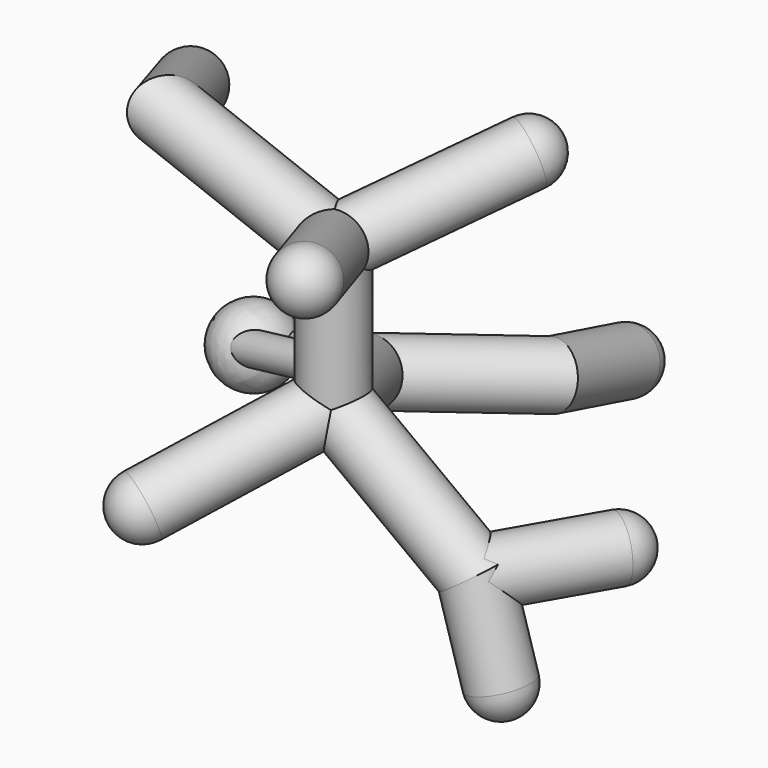
from build123d import *

# Parameters (mm, degrees)
F9_R  = 6
F13_R = 6
F18_R = 6
F26_R = 6
F29_R = 6
F31_R = 6
F34_R = 3


with BuildPart() as f11:
    # F11: sweep along a path in F7, F4
    with BuildLine(Plane(origin=(-5.0749581016, 8.7900852782, 27.9244028222), x_dir=(0.9853046871, 0.051285676, 0.1629246852), z_dir=(0.1708059531, -0.295844589, -0.9398411066))) as f11_path:
        Line((2.0467480645, -75.1046538353), (6.1499904841, -45.6850528717))
        Line((6.1499904841, -45.6850528717), (-12.6624797904, -23.3359215656))
        Line((-12.6624797904, -23.3359215656), (5.1506484929, 9.4922267384))
    with BuildLine(Plane.XZ) as f11_path_2:
        Line((0, 31.6136777401), (0, 58.9116849005))
    # F9 (on line) → F11 (sweep)
    with BuildSketch(Plane(origin=(-10.0857183749, 69.480148269, -23.7040351701), x_dir=(-0.9906942747, -0.1288157724, 0.0439471371), z_dir=(-0.1361060398, 0.9376295745, -0.3198842398))):
        with Locations((-7.0934403418, 31.4051011688)):
            Circle(F9_R)
    sweep(path=f11_path.line + f11_path_2.line, transition=Transition.RIGHT)

    # F14: sweep along a path in F4, F10
    with BuildLine(Plane.XZ) as f14_path:
        Line((34.7157008946, -12.1698062867), (27.8801377863, 10.8416592702))
        Line((27.8801377863, 10.8416592702), (0, 31.6136777401))
    with BuildLine(Plane(origin=(0, 0, 0), x_dir=(-0.5, -0.8660254038, 0), z_dir=(-0.8660254038, 0.5, 0))) as f14_path_2:
        Line((0, 31.6136777401), (37.2237116098, 17.5120830536))
    # F13 (on line) → F14 (sweep)
    with BuildSketch(Plane(origin=(6.1368140533, 0, -20.6591736452), x_dir=(0.9586010028, 0, 0.2847527305), z_dir=(0.2847527305, 0, -0.9586010028))):
        with Locations((29.8131201191, 0)):
            Circle(F13_R)
    sweep(path=f14_path.line + f14_path_2.line, transition=Transition.RIGHT)

    # F19: sweep along a path in F16
    with BuildLine(Plane.XY.offset(10.8416592702)) as f19_path:
        Line((27.8801377863, 0), (42.7882038549, 25.8215278734))
    # F18 (on line) → F19 (sweep)
    with BuildSketch(Plane(origin=(21.8781005152, 37.8939816654, 0), x_dir=(-0.8660254038, 0.5, 0), z_dir=(0.5, 0.8660254038, 0))):
        with Locations((-24.1449075839, 10.8416592702)):
            Circle(F18_R)
    sweep(path=f19_path.line)

    # F27: sweep along a path in F27_path
    with BuildLine(Plane(origin=(0, 0, 58.9116849005), x_dir=(0.8527843216, 0, 0.5222632486), z_dir=(0.5222626897, 0.0014629567, -0.852783409))) as f27_path:
        Line((20.2068447746, 29.8864215955), (0, 0))
        Line((0, 0), (22.3578653078, -32.9804275589))
    # F26 (on line) → F27 (sweep)
    with BuildSketch(Plane(origin=(25.4681834782, -44.1121877608, 15.5215822052), x_dir=(0.8782037706, 0.4511717321, -0.1587520249), z_dir=(0.4782866685, -0.8284168104, 0.2914917685))):
        with Locations((-9.352349266, 55.5718749217)):
            Circle(F26_R)
    sweep(path=f27_path.line, transition=Transition.RIGHT)

    # F30: sweep along a path in F30_path
    with BuildLine(Plane(origin=(-32.6037183404, 0, 71.4510455728), x_dir=(0, -0.8308020039, 0.5565680824), z_dir=(-0.3043658699, -0.5301618235, -0.7913847725))) as f30_path:
        Line((-32.401113983, 19.9450910541), (0, 0))
        Line((0, 0), (-6.979007924, -34.2276418131))
    # F29 (on line) → F30 (sweep)
    with BuildSketch(Plane(origin=(-14.9472358293, 23.8365368187, -10.2197991039), x_dir=(-0.8664063143, -0.4589367006, 0.1967668759), z_dir=(-0.4993396626, 0.7963029678, -0.3414110204))):
        with Locations((42.3072664543, 65.6697425993)):
            Circle(F29_R)
    sweep(path=f30_path.line, transition=Transition.RIGHT)

    # F31
    f31_edges = [f11.edges().sort_by_distance(p)[0] for p in [
        (28.964095, 0, -13.878323),
        (2.885878, 81.30715, 5.443491),
        (-18.507369, -29.883149, 11.993933),
        (47.984356, 22.821528, 10.841659),
        (13.770717, 35.68189, 71.590517),
        (-46.404081, 33.051236, 57.280489),
        (11.985692, -32.59342, 70.380204),
    ]]
    fillet(f31_edges, radius=F31_R)

    # F35: sweep along a path in F32
    with BuildLine(Plane(origin=(-5.0749581016, 8.7900852782, 27.9244028222), x_dir=(0.9853046871, 0.051285676, 0.1629246852), z_dir=(0.1708059531, -0.295844589, -0.9398411066))) as f35_path:
        Line((-12.6624797904, -23.3359215656), (-41.0683602095, -32.030723989))
    # F34 (on line) → F35 (sweep)
    with BuildSketch(Plane(origin=(-45.8310956024, 11.1952553321, -11.8533649983), x_dir=(-0.2228111413, -0.9731569461, -0.0576259797), z_dir=(-0.9421564229, 0.2301424738, -0.2436713288))):
        with Locations((-23.1341181113, 24.1245243578)):
            Circle(F34_R)
        with Locations((-29.9624393627, 21.6161606898)):
            Circle(F34_R)
    sweep(path=f35_path.line)

    # F36 (on face) → F37 (revolve)
    with BuildSketch(Plane(origin=(-5.0749581016, 8.7900852782, 27.9244028222), x_dir=(0.9853046871, 0.051285676, 0.1629246852), z_dir=(0.1708059531, -0.295844589, -0.9398411066))):
        with BuildLine():
            Line((-33.8562362695, -29.4675207461), (-48.0667891911, -34.1731258904))
            ThreePointArc((-48.0667891911, -34.1731258904), (-38.6087101581, -38.925599779), (-33.8562362695, -29.4675207461))
        make_face()
    revolve(axis=Axis((-45.4345285849, 37.041427616, 11.6964877452), (-0.9353572599, 0.2511581183, -0.2490509905)))


solid = f11.part
